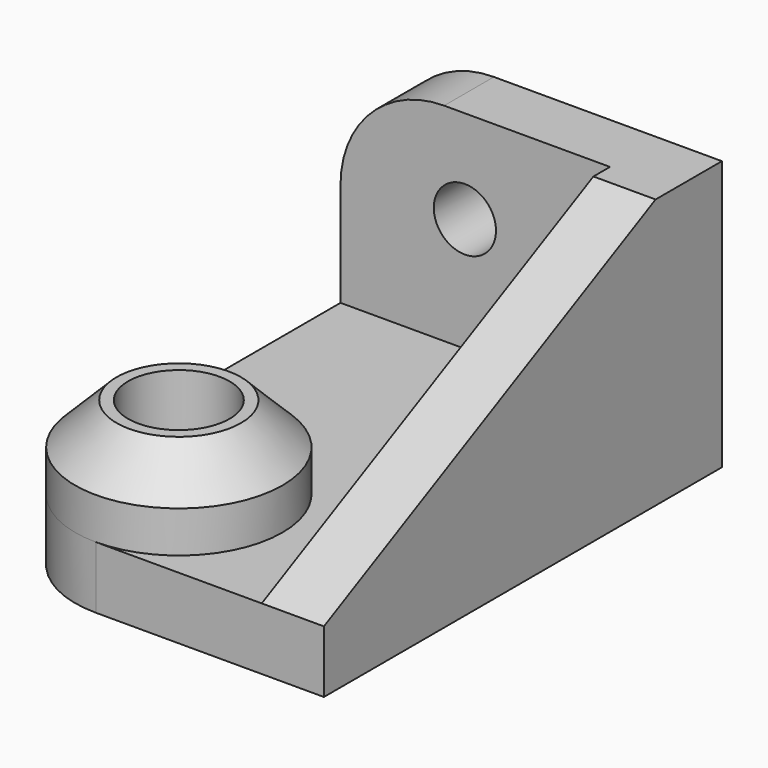
from build123d import *

# Parameters (mm, degrees)
F0_W     = 16
F0_H     = 24
F1_DEPTH = 13
F2_T     = -3
F3_R     = 5
F4_DEPTH = 4
F5_D     = 4.9
F6_SIZE2 = 10
F6_SIZE  = 20
F7_R     = 5
F8_SIZE  = 2
F10_D    = 3
F11_R    = 4.9999


# Not quite as in the source:
# - a fillet or chamfer is up to 0.001 mm smaller than in the source, because OpenCascade refuses the exact size


with BuildPart() as f1:
    # F0 (on Top) → F1 (new body)
    with BuildSketch(Plane.XY):
        with Locations((8, 12)):
            Rectangle(F0_W, F0_H)
    extrude(amount=F1_DEPTH)

    # F2
    f2_openings = [f1.faces().sort_by_distance(p)[0] for p in [
        (8, 0, 6.5),
        (0, 12, 6.5),
        (8, 12, 13),
    ]]
    offset(amount=F2_T, openings=f2_openings)

    # F3 (on face) → F4 (join)
    with BuildSketch(Plane.XY.offset(3)):
        with Locations((5, 5)):
            Circle(F3_R)
    extrude(amount=F4_DEPTH)

    # F5 (through all)
    with Locations(Plane(origin=(0, 0, 0), x_dir=(1, 0, 0), z_dir=(0, 0, -1))):
        with Locations((5, -5)):
            Hole(F5_D / 2)

    # F6
    f6_edges = [f1.edges().sort_by_distance(p)[0] for p in [
        (14.5, 0, 13),
    ]]
    f6_side = f1.faces().sort_by_distance((8, 23.711556, 13))[0]
    chamfer(f6_edges, length=F6_SIZE, length2=F6_SIZE2, reference=f6_side)

    # F7
    f7_edges = [f1.edges().sort_by_distance(p)[0] for p in [
        (0, 22.5, 13),
    ]]
    fillet(f7_edges, radius=F7_R)

    # F8
    f8_edges = [f1.edges().sort_by_distance(p)[0] for p in [
        (0, 5, 7),
    ]]
    chamfer(f8_edges, length=F8_SIZE)

    # F10 (through all)
    with Locations(Plane(origin=(0, 24, 0), x_dir=(-1, 0, 0), z_dir=(0, 1, 0))):
        with Locations((-6, 8.5)):
            Hole(F10_D / 2)

    # F11 (radius 5 in the source; OpenCascade refuses exactly that, so slightly less here)
    f11_edges = [f1.edges().sort_by_distance(p)[0] for p in [
        (0, 0, 1.5),
    ]]
    fillet(f11_edges, radius=F11_R)


solid = f1.part
